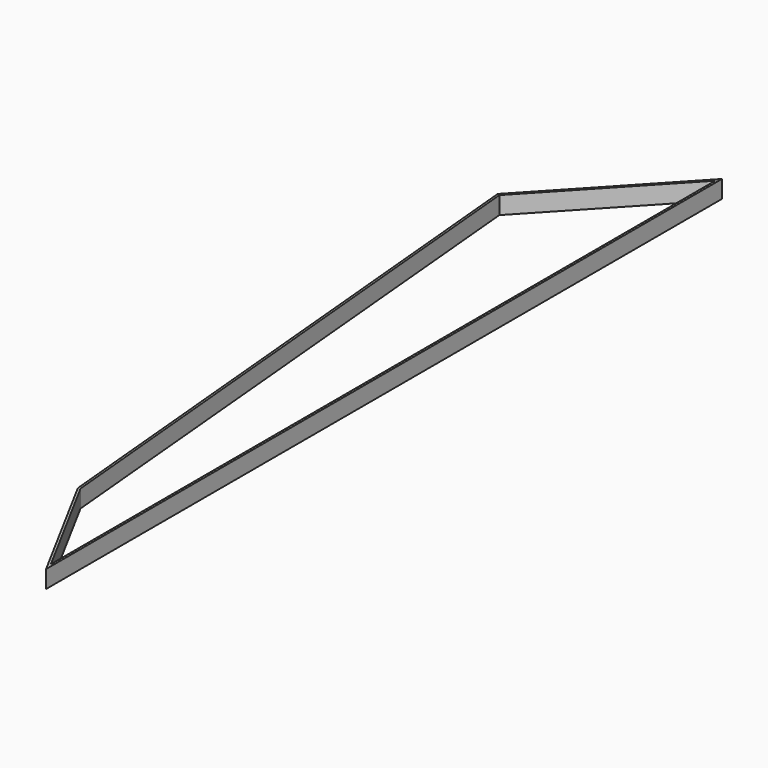
from build123d import *

# Parameters (mm, degrees)
F1_DEPTH = 25.4


# Not quite as in the source:
# - the program builds the solid bodies; features that only make, move or delete a surface that nothing else refers to are left out


with BuildPart() as f1:
    # F0 (on Top) → F1 (new body)
    with BuildSketch(Plane.XY):
        Polygon((-95.5357477069, 176.7154484987), (0, 0), (0, 1219.2), (-174.515992403, 1032.7594280243), align=None)
        Polygon((-171.2233918284, 1031.6309448815), (-3.175, 1211.1619887742), (-3.175, 12.5490882171), (-92.4338527853, 177.6539686524), align=None, mode=Mode.SUBTRACT)
    extrude(amount=F1_DEPTH)


solid = f1.part
